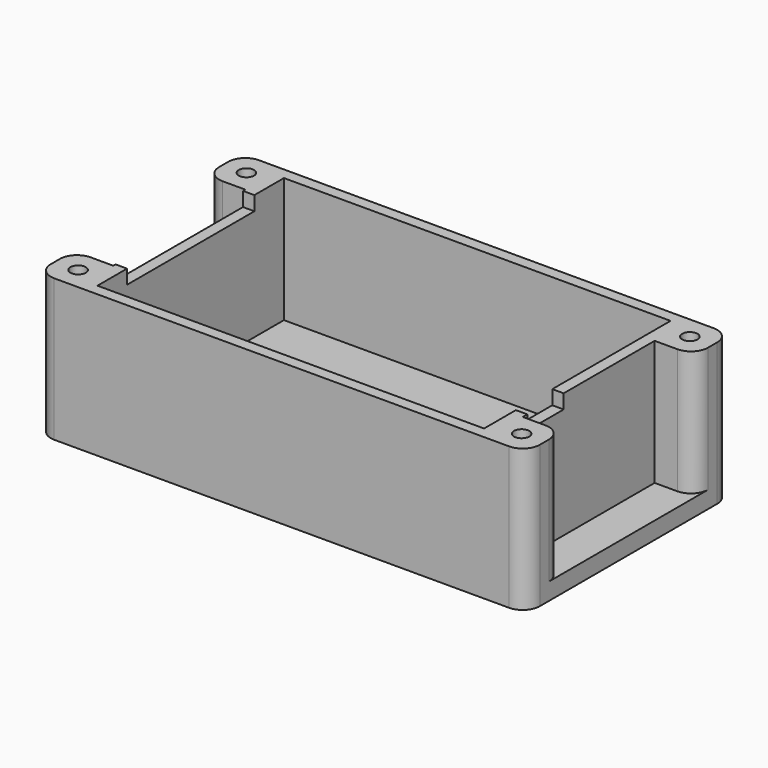
from build123d import *

# Parameters (mm, degrees)
F0_W     = 86
F0_H     = 45
F1_DEPTH = 3
F2_R     = 1.35
F2_W     = 68
F2_H     = 41
F3_DEPTH = 22
F4_R     = 3
F5_W     = 2
F5_H     = 28
F5_H_2   = 8
F6_DEPTH = 2.5


# Not quite as in the source:
# - a feature names something its author has since deleted; it is built from what else it names


with BuildPart() as f1:
    # F0 (on Top) → F1 (new body)
    with BuildSketch(Plane.XY):
        Rectangle(F0_W, F0_H)
    extrude(amount=F1_DEPTH)

    # F2 (on face) → F3 (join)
    with BuildSketch(Plane.XY.offset(3)):
        Polygon((43, 22.5), (-43, 22.5), (-43, 14.5), (-36, 14.5), (-36, -14.5), (-43, -14.5), (-43, -22.5), (43, -22.5), (43, -14.5), (36, -14.5), (36, 14.5), (43, 14.5), align=None)
        with Locations((-39, -18.5)):
            Circle(F2_R, mode=Mode.SUBTRACT)
        with Locations((39, -18.5)):
            Circle(F2_R, mode=Mode.SUBTRACT)
        with Locations((-39, 18.5)):
            Circle(F2_R, mode=Mode.SUBTRACT)
        Rectangle(F2_W, F2_H, mode=Mode.SUBTRACT)
        with Locations((39, 18.5)):
            Circle(F2_R, mode=Mode.SUBTRACT)
    extrude(amount=F3_DEPTH)

    # F4
    f4_edges = [f1.edges().sort_by_distance(p)[0] for p in [
        (-43, -22.5, 12.5),
        (-43, 14.5, 14),
        (-43, 22.5, 12.5),
        (-43, -14.5, 14),
        (43, -22.5, 12.5),
        (43, -14.5, 14),
        (43, 14.5, 14),
        (43, 22.5, 12.5),
    ]]
    fillet(f4_edges, radius=F4_R)

    # F5 (on face) → F6 (cut)
    with BuildSketch(Plane.XY.offset(25)):
        with Locations((-35, 0)):
            Rectangle(F5_W, F5_H)
        with Locations((35, -9.5)):
            Rectangle(F5_W, F5_H_2)
    extrude(amount=-F6_DEPTH, mode=Mode.SUBTRACT)


solid = f1.part
